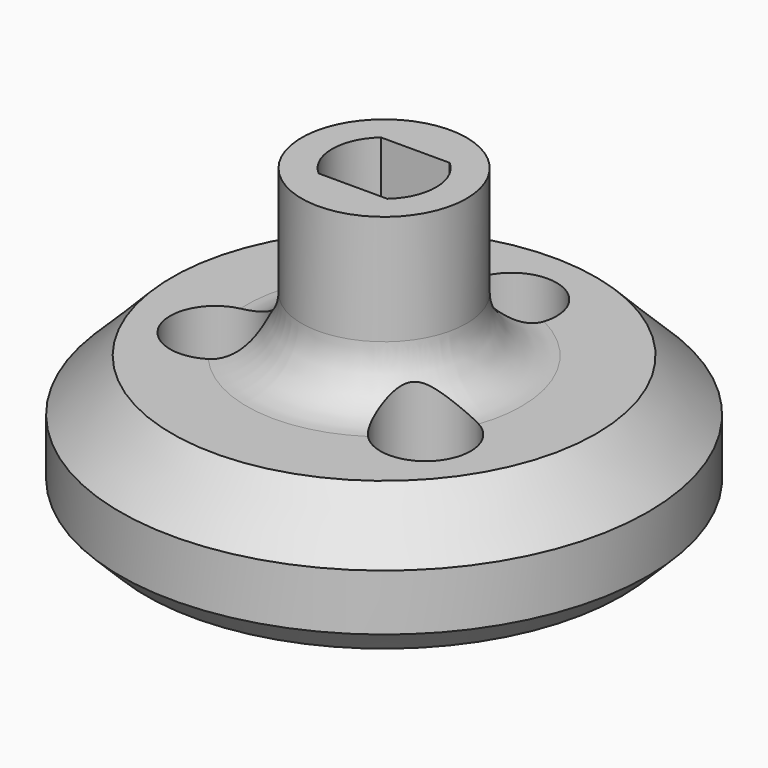
from build123d import *

# Parameters (mm, degrees)
F0_R          = 4.7625
F1_DEPTH      = 9.525
F1_DEPTH_BACK = 6.35
F3_DEPTH      = 9.526
F4_R          = 15.24
F5_DEPTH      = 7.75
F6_R          = 2.6035
F7_DEPTH      = 13.97
F8_SIZE       = 1.5
F9_SIZE       = 3
F10_S5_R      = 2.6035
F10_T6_DEPTH  = 14
F10_S7_R      = 2.6035
F10_T8_DEPTH  = 14
F10_S9_R      = 2.6035
F10_T10_DEPTH = 14


# Not quite as in the source:
# - a fillet or chamfer that OpenCascade refuses, or shapes differently, is made with other operations: its cross-section is extruded or revolved along the edge and cut away or added


with BuildPart() as f1:
    # F0 (on Top) → F1 (new body, two sides)
    with BuildSketch(Plane.XY) as f1_sk:
        Circle(F0_R)
    extrude(amount=F1_DEPTH)
    extrude(f1_sk.sketch, amount=-F1_DEPTH_BACK)

    # F2 (on Top) → F3 (cut, through all)
    with BuildSketch(Plane.XY):
        with BuildLine():
            ThreePointArc((1.9843134833, -2.25), (2.7343134833, -1.2343134833), (3, 0))
            ThreePointArc((3, 0), (2.7343134833, 1.2343134833), (1.9843134833, 2.25))
            Line((1.9843134833, 2.25), (-1.9843134833, 2.25))
            ThreePointArc((-1.9843134833, 2.25), (-3, 0), (-1.9843134833, -2.25))
            Line((-1.9843134833, -2.25), (1.9843134833, -2.25))
        make_face()
    extrude(amount=F3_DEPTH, mode=Mode.SUBTRACT)

    # F4 (on Top) → F5 (join)
    with BuildSketch(Plane.XY):
        Circle(F4_R)
    extrude(amount=-F5_DEPTH)

    # F6 (on face) → F7 (cut)
    with BuildSketch(Plane(origin=(0, 0, -7.75), x_dir=(1, 0, 0), z_dir=(0, 0, -1))):
        with Locations((1.0674559099, -7.8653953575)):
            Circle(F6_R)
        with Locations((6.2779042355, 4.8571416142)):
            Circle(F6_R)
        with Locations((-7.3453601454, 3.0082537434)):
            Circle(F6_R)
    extrude(amount=-F7_DEPTH, mode=Mode.SUBTRACT)

    # F8
    f8_edges = [f1.edges().sort_by_distance(p)[0] for p in [
        (-15.24, 0, -7.75),
    ]]
    chamfer(f8_edges, length=F8_SIZE)

    # F9
    f9_edges = [f1.edges().sort_by_distance(p)[0] for p in [
        (-15.24, 0, 0),
    ]]
    chamfer(f9_edges, length=F9_SIZE)

    # F10: fillet of radius 3.175 on 1 edges, made by hand


with BuildPart() as f10_tool2:
    # F10_s3 → F10_t4 (revolve)
    with BuildSketch(Plane.XZ):
        with BuildLine():
            ThreePointArc((7.9375, 0), (5.6924359697, 0.9299359697), (4.7625, 3.175))
            Line((4.7625, 3.175), (4.7625, 0))
            Line((4.7625, 0), (7.9375, 0))
        make_face()
    revolve(axis=Axis((0, 0, 0), (0, 0, 1)))

    # F10_s5 → F10_t6 (cut, symmetric)
    with BuildSketch(Plane.XY.offset(2.7)):
        with Locations((-7.3453601454, -3.0082537434)):
            Circle(F10_S5_R)
    extrude(amount=F10_T6_DEPTH, both=True, mode=Mode.SUBTRACT)

    # F10_s7 → F10_t8 (cut, symmetric)
    with BuildSketch(Plane.XY.offset(2.7)):
        with Locations((6.2779042355, -4.8571416142)):
            Circle(F10_S7_R)
    extrude(amount=F10_T8_DEPTH, both=True, mode=Mode.SUBTRACT)

    # F10_s9 → F10_t10 (cut, symmetric)
    with BuildSketch(Plane.XY.offset(2.7)):
        with Locations((1.0674559099, 7.8653953575)):
            Circle(F10_S9_R)
    extrude(amount=F10_T10_DEPTH, both=True, mode=Mode.SUBTRACT)


with BuildPart() as f1_1:
    add(f1.part)

    # F10_t1: union F10_tool2
    add(f10_tool2.part)


solid = f1_1.part
